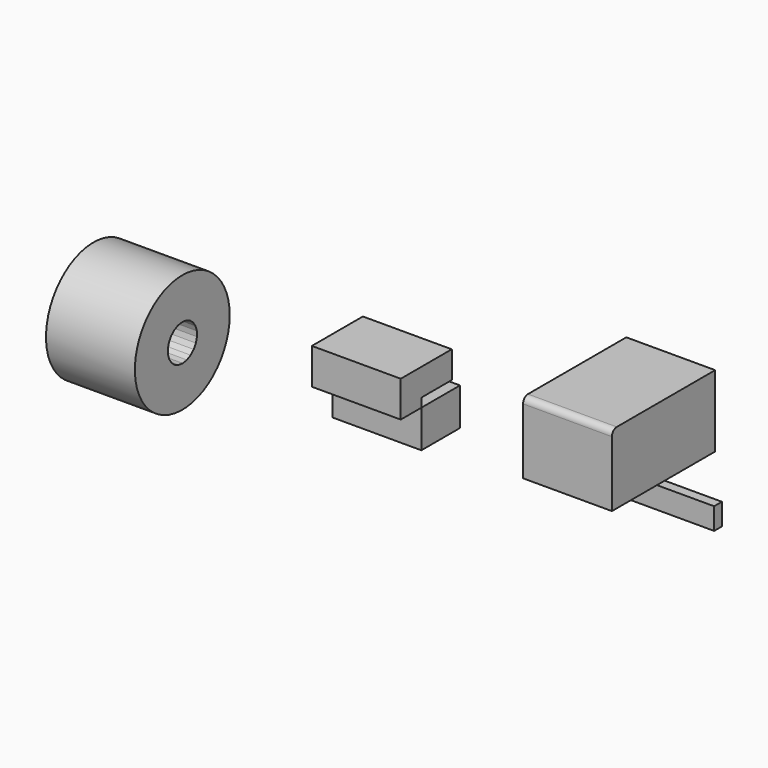
from build123d import *

# Parameters (mm, degrees)
F0_W     = 50.2453520894
F0_H     = 39.0470791608
F1_DEPTH = 92.456
F0_W_2   = 26.8350038677
F0_H_2   = 9.2546753585
F0_W_3   = 39.5157057792
F0_H_3   = 28.1695313752
F0_W_4   = 3.8517713547
F0_H_4   = 74.5441019535
F0_W_5   = 10.1218819618
F0_H_5   = 22.6000696421
F0_R     = 61.6690599932


with BuildPart() as f1:
    # F0 (on Right) → F1 (new body)
    with BuildSketch(Plane.YZ):
        with Locations((6.0294363648, 2.2069280967)):
            Rectangle(F0_W, F0_H)
    extrude(amount=F1_DEPTH)


with BuildPart() as f1b:
    # F0 (on Right) → F1, piece 2 (new body)
    with BuildSketch(Plane.YZ):
        with Locations((-32.5107416138, 26.3578053564)):
            Rectangle(F0_W_2, F0_H_2)
        with Locations((0.6646132097, 45.0699087232)):
            Rectangle(F0_W_3, F0_H_3)
        with Locations((-32.5107416138, 45.0699087232)):
            Rectangle(F0_W_2, F0_H_3)
    extrude(amount=F1_DEPTH)


with BuildPart() as f1c:
    # F0 (on Right) → F1, piece 3 (new body)
    with BuildSketch(Plane.YZ):
        with Locations((361.0702455044, -136.4756524563)):
            Rectangle(F0_W_4, F0_H_4)
        with BuildLine():
            Line((228.7123948336, -173.747703433), (359.144359827, -173.747703433))
            Line((359.144359827, -173.747703433), (359.144359827, -99.2036014795))
            Line((359.144359827, -99.2036014795), (235.0623948336, -99.2036014795))
            ThreePointArc((235.0623948336, -99.2036014795), (230.572266773, -101.063473419), (228.7123948336, -105.5536014795))
            Line((228.7123948336, -105.5536014795), (228.7123948336, -173.747703433))
        make_face()
    extrude(amount=F1_DEPTH)


with BuildPart() as f1d:
    # F0 (on Right) → F1, piece 4 (new body)
    with BuildSketch(Plane.YZ):
        with Locations((366.7074739933, -234.6265390515)):
            Rectangle(F0_W_5, F0_H_5)
    extrude(amount=F1_DEPTH)


with BuildPart() as f1e:
    # F0 (on Right) → F1, piece 5 (new body)
    with BuildSketch(Plane.YZ):
        with Locations((-330.0160169601, 207.8216075897)):
            Circle(F0_R)
        Polygon((-348.6337553052, 204.3390901534), (-348.7787469344, 209.7568042641), (-347.3915189352, 214.9959117489), (-344.5844562699, 219.6319712773), (-340.5849704614, 223.2893968782), (-335.7170760642, 225.671885681), (-330.3751409316, 226.5864226119), (-324.9919368786, 225.9589173279), (-320.0035790823, 223.8402065751), (-315.8141946244, 220.4019356983), (-312.7631825185, 215.9226529557), (-311.0977176204, 210.7652431959), (-310.9527259912, 205.3475290851), (-312.3399539904, 200.1084216004), (-315.1470166557, 195.4723620719), (-319.1465024641, 191.814936471), (-324.0143968614, 189.4324476683), (-329.3563319939, 188.5179107373), (-334.739536047, 189.1454160213), (-339.7278938433, 191.2641267741), (-343.9172783012, 194.7023976509), (-346.9682904071, 199.1816803935), align=None, mode=Mode.SUBTRACT)
    extrude(amount=F1_DEPTH)


solid = Compound([f1.part, f1b.part, f1c.part, f1d.part, f1e.part])
